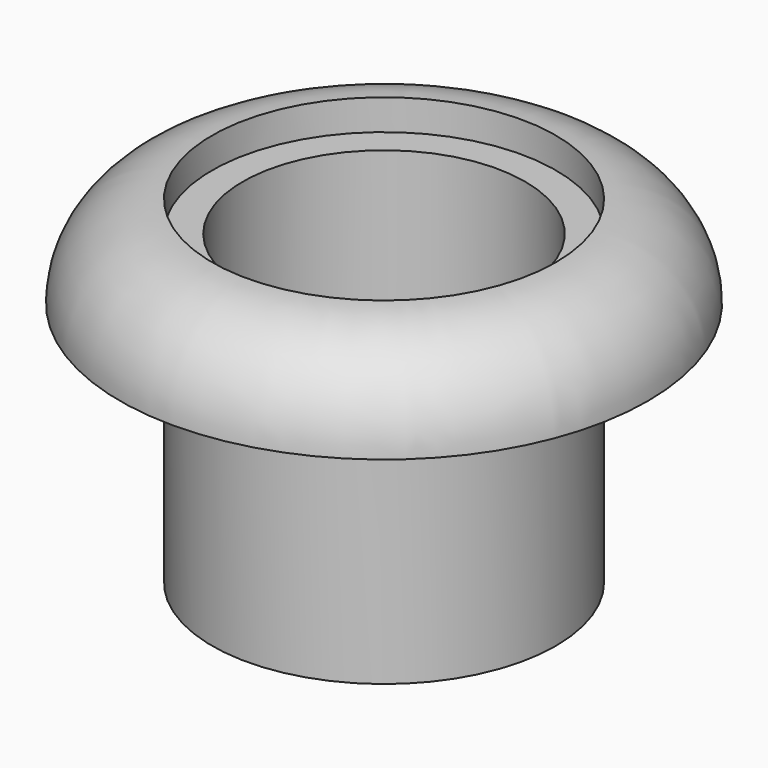
from build123d import *

# Parameters (mm, degrees)
F2_R     = 14.99999
F4_D     = 5
F5_R     = 28
F5_R_2   = 23
F6_DEPTH = 5


# Not quite as in the source:
# - a fillet or chamfer is up to 0.001 mm smaller than in the source, because OpenCascade refuses the exact size


with BuildPart() as f1:
    # F0 (on Front) → F1 (revolve)
    with BuildSketch(Plane.XZ):
        Polygon((43, 15), (43, 30), (23, 30), (23, -20), (0, -20), (0, -25), (28, -25), (28, -15), (28, 15), align=None)
    revolve(axis=Axis((0, 0, -22.5), (0, 0, -1)))

    # F2 (radius 15 in the source; OpenCascade refuses exactly that, so slightly less here)
    f2_edges = [f1.edges().sort_by_distance(p)[0] for p in [
        (-43, 0, 30),
    ]]
    fillet(f2_edges, radius=F2_R)

    # F4 (through all)
    with Locations(Plane.XY.offset(-20)):
        with Locations((0, 15), (-12.9903810568, -7.5), (12.9903810568, -7.5)):
            Hole(F4_D / 2)

    # F5 (on face) → F6 (cut)
    with BuildSketch(Plane.XY.offset(30)):
        Circle(F5_R)
        Circle(F5_R_2, mode=Mode.SUBTRACT)
    extrude(amount=-F6_DEPTH, mode=Mode.SUBTRACT)


solid = f1.part
